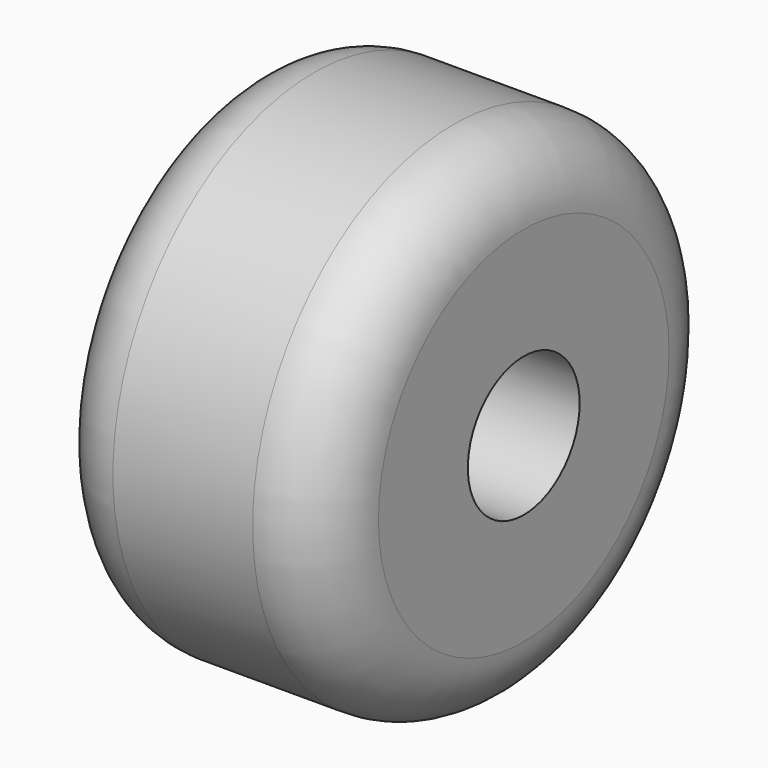
from build123d import *

# Parameters (mm, degrees)
F0_R     = 18
F1_DEPTH = 20
F2_R     = 5
F3_DEPTH = 15
F4_R     = 5
F5_R     = 13
F6_DEPTH = 2
F7_SIZE  = 1.99999


# Not quite as in the source:
# - a fillet or chamfer is up to 0.001 mm smaller than in the source, because OpenCascade refuses the exact size


with BuildPart() as f1:
    # F0 (on Right) → F1 (new body)
    with BuildSketch(Plane.YZ):
        Circle(F0_R)
    extrude(amount=F1_DEPTH)

    # F2 (on face) → F3 (cut)
    with BuildSketch(Plane.YZ.offset(20)):
        Circle(F2_R)
    extrude(amount=-F3_DEPTH, mode=Mode.SUBTRACT)

    # F4
    f4_edges = [f1.edges().sort_by_distance(p)[0] for p in [
        (0, -18, 0),
        (20, -18, 0),
    ]]
    fillet(f4_edges, radius=F4_R)

    # F5 (on face) → F6 (cut)
    with BuildSketch(Plane(origin=(0, 0, 0), x_dir=(0, -1, 0), z_dir=(-1, 0, 0))):
        Circle(F5_R)
    extrude(amount=-F6_DEPTH, mode=Mode.SUBTRACT)

    # F7 (size 2 in the source; OpenCascade refuses exactly that, so slightly less here)
    f7_edges = [f1.edges().sort_by_distance(p)[0] for p in [
        (2, 13, 0),
    ]]
    chamfer(f7_edges, length=F7_SIZE)


solid = f1.part
